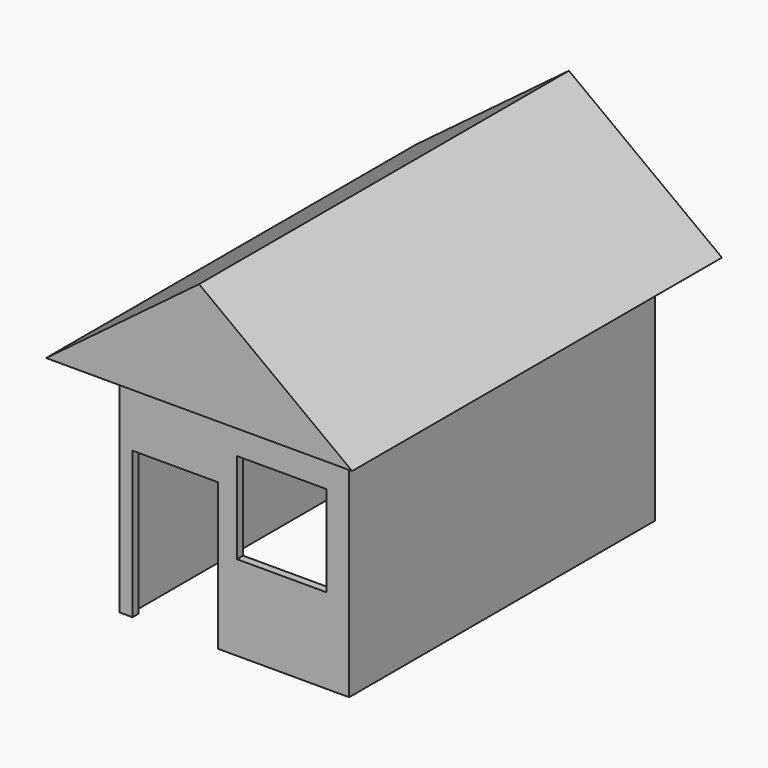
from build123d import *

# Parameters (mm, degrees)
F0_W          = 76.2
F0_H          = 76.2
F1_DEPTH      = 127
F3_DEPTH      = 14.65342
F3_DEPTH_BACK = 138.81125
F4_T          = -2.54
F6_W          = 29.8130884767
F6_H          = 30.159747228
F6_W_2        = 28.4264292568
F6_H_2        = 48.6897528172
F7_DEPTH      = 25.4


with BuildPart() as f1:
    # F0 (on Front) → F1 (new body)
    with BuildSketch(Plane.XZ):
        with Locations((38.1, 38.1)):
            Rectangle(F0_W, F0_H)
    extrude(amount=-F1_DEPTH)

    # F2 (on Front) → F3 (join, two sides)
    with BuildSketch(Plane.XZ) as f3_sk:
        Polygon((38.1, 114.3), (38.1, 76.2), (76.2, 76.2), (88.9, 76.2), align=None)
        Polygon((-12.7, 76.2), (0, 76.2), (38.1, 76.2), (38.1, 114.3), align=None)
    extrude(amount=F3_DEPTH)
    extrude(f3_sk.sketch, amount=-F3_DEPTH_BACK)

    # F4
    f4_openings = [f1.faces().sort_by_distance(p)[0] for p in [
        (38.1, 63.5, 0),
    ]]
    offset(amount=F4_T, openings=f4_openings, kind=Kind.INTERSECTION)

    # F6 (on Front) → F7 (cut)
    with BuildSketch(Plane.XZ):
        with Locations((53.8429357111, 43.3164620772)):
            Rectangle(F6_W, F6_H)
        with Locations((18.4832299128, 24.3448764086)):
            Rectangle(F6_W_2, F6_H_2)
    extrude(amount=-F7_DEPTH, mode=Mode.SUBTRACT)


solid = f1.part
